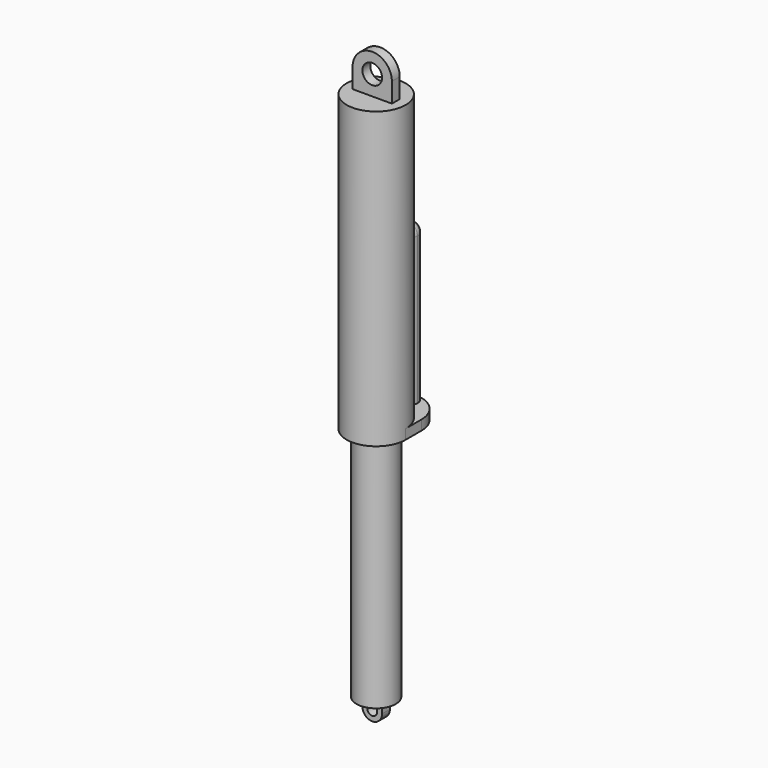
from build123d import *

# Parameters (mm, degrees)
F0_R         = 38.1
F1_DEPTH     = 381
F2_R         = 25.4
F3_DEPTH     = 304.8
F4_W         = 38.1
F4_H         = 63.5
F5_DEPTH     = 12.7
F7_DEPTH     = 203.2
F8_R         = 38.09999
F9_T3_ANGLE  = 359.64
F9_S4_R      = 38.1
F9_T5_DEPTH  = 21
F9_T8_ANGLE  = 230.2151920397
F9_S9_R      = 38.1
F9_T10_DEPTH = 20
F10_W        = 50.8
F10_H        = 12.7
F11_DEPTH    = 25.4
F13_DEPTH    = 12.7
F15_D        = 25.4
F16_W        = 25.4
F16_H        = 12.7
F17_DEPTH    = 12.7
F19_DEPTH    = 12.7
F21_D        = 12.7


# Not quite as in the source:
# - a fillet or chamfer that OpenCascade refuses, or shapes differently, is made with other operations: its cross-section is extruded or revolved along the edge and cut away or added
# - a fillet or chamfer is up to 0.001 mm smaller than in the source, because OpenCascade refuses the exact size


with BuildPart() as f1:
    # F0 (on Top) → F1 (new body)
    with BuildSketch(Plane.XY):
        Circle(F0_R)
    extrude(amount=F1_DEPTH)

    # F2 (on Top) → F3 (join)
    with BuildSketch(Plane.XY):
        Circle(F2_R)
    extrude(amount=-F3_DEPTH)

    # F4 (on Top) → F5 (join)
    with BuildSketch(Plane.XY):
        with Locations((19.05, 31.75)):
            Rectangle(F4_W, F4_H)
        with Locations((-19.05, 31.75)):
            Rectangle(F4_W, F4_H)
    extrude(amount=F5_DEPTH)

    # F6 (on face) → F7 (join)
    with BuildSketch(Plane.XY.offset(12.7)):
        with BuildLine():
            ThreePointArc((0.6819155813, 38.0938970327), (9.2181974345, 42.0397400715), (12.7, 50.7755763829))
            ThreePointArc((12.7, 50.7755763829), (-8.7358363114, 59.9937738174), (-0.6819155813, 38.0938970327))
            ThreePointArc((-0.6819155813, 38.0938970327), (0, 38.1), (0.6819155813, 38.0938970327))
        make_face()
        with BuildLine():
            ThreePointArc((0.6819155813, 38.0938970327), (0, 38.1), (-0.6819155813, 38.0938970327))
            ThreePointArc((-0.6819155813, 38.0938970327), (0, 38.0755763829), (0.6819155813, 38.0938970327))
        make_face()
    extrude(amount=F7_DEPTH)

    # F8 (radius 38.1 in the source; OpenCascade refuses exactly that, so slightly less here)
    f8_edges = [f1.edges().sort_by_distance(p)[0] for p in [
        (-38.1, 63.5, 6.35),
        (38.1, 63.5, 6.35),
    ]]
    fillet(f8_edges, radius=F8_R)

    # F9: fillet of radius 12.7 on 2 edges, made by hand


with BuildPart() as f9_tool1:
    # F9_s2 → F9_t3 (revolve)
    with BuildSketch(Plane.XZ.offset(-50.7755763829)):
        with BuildLine():
            ThreePointArc((0, 215.9), (8.9802561211, 212.1802561211), (12.7, 203.2))
            Line((12.7, 203.2), (12.7, 215.9))
            Line((12.7, 215.9), (0, 215.9))
        make_face()
    revolve(axis=Axis((0, 50.7755763829, 215.9), (0, 0, 1)), revolution_arc=F9_T3_ANGLE)

    # F9_s4 → F9_t5 (cut, symmetric)
    with BuildSketch(Plane.XY.offset(209.5)):
        Circle(F9_S4_R)
    extrude(amount=F9_T5_DEPTH, both=True, mode=Mode.SUBTRACT)


with BuildPart() as f9_tool6:
    # F9_s7 → F9_t8 (revolve)
    with BuildSketch(Plane(origin=(24.9682702957, 20.7915649924, 0), x_dir=(0, 0, 1), z_dir=(0.7684532224, 0.6399059658, 0))):
        with BuildLine():
            ThreePointArc((203.2, -51.7186552898), (212.1802561211, -47.9989114109), (215.9, -39.0186552898))
            Line((215.9, -39.0186552898), (215.9, -51.7186552898))
            Line((215.9, -51.7186552898), (203.2, -51.7186552898))
        make_face()
    revolve(axis=Axis((0, 50.7755763829, 215.9), (0, 0, 1)), revolution_arc=F9_T8_ANGLE)

    # F9_s9 → F9_t10 (cut, symmetric)
    with BuildSketch(Plane.XY.offset(209.5)):
        Circle(F9_S9_R)
    extrude(amount=F9_T10_DEPTH, both=True, mode=Mode.SUBTRACT)


with BuildPart() as f1_1:
    add(f1.part)

    # F9_t11: cut F9_tool1, F9_tool6
    add([f9_tool1.part, f9_tool6.part], mode=Mode.SUBTRACT)

    # F10 (on face) → F11 (join)
    with BuildSketch(Plane.XY.offset(381)):
        Rectangle(F10_W, F10_H)
    extrude(amount=F11_DEPTH)

    # F12 (on face) → F13 (join)
    with BuildSketch(Plane(origin=(0, 6.35, 0), x_dir=(-1, 0, 0), z_dir=(0, 1, 0))):
        with BuildLine():
            Line((-25.4, 406.4), (25.4, 406.4))
            ThreePointArc((25.4, 406.4), (0, 431.8), (-25.4, 406.4))
        make_face()
    extrude(amount=-F13_DEPTH)

    # F15 (through all)
    with Locations(Plane(origin=(0, 6.35, 0), x_dir=(-1, 0, 0), z_dir=(0, 1, 0))):
        with Locations((0, 406.4)):
            Hole(F15_D / 2)

    # F16 (on face) → F17 (join)
    with BuildSketch(Plane(origin=(0, 0, -304.8), x_dir=(1, 0, 0), z_dir=(0, 0, -1))):
        Rectangle(F16_W, F16_H)
    extrude(amount=F17_DEPTH)

    # F18 (on face) → F19 (join)
    with BuildSketch(Plane.XZ.offset(6.35)):
        with BuildLine():
            Line((12.7, -317.5), (-12.7, -317.5))
            ThreePointArc((-12.7, -317.5), (0, -330.2), (12.7, -317.5))
        make_face()
    extrude(amount=-F19_DEPTH)

    # F21 (through all)
    with Locations(Plane.XZ.offset(6.35)):
        with Locations((0, -317.5)):
            Hole(F21_D / 2)


solid = f1_1.part
